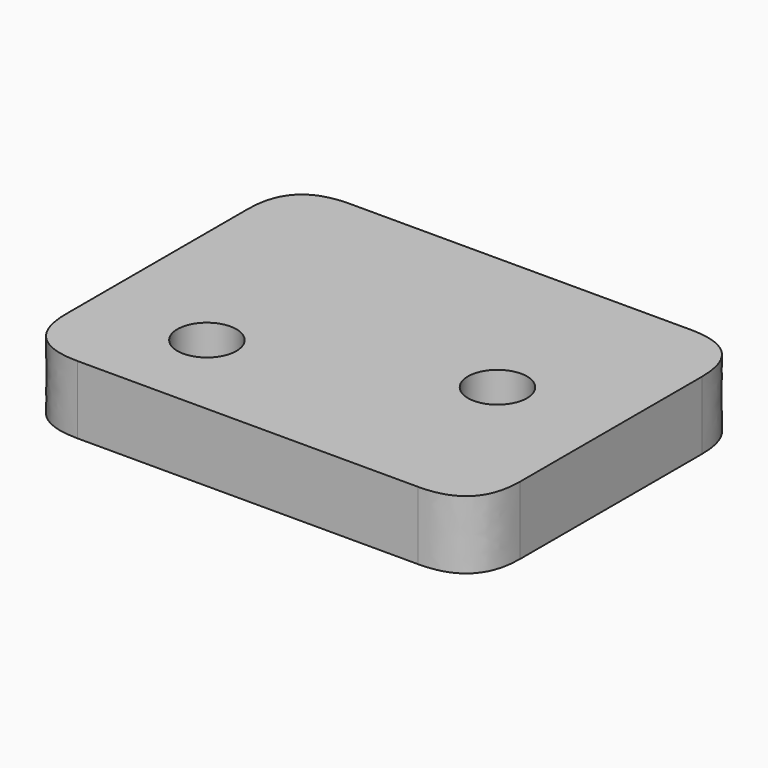
from build123d import *

# Parameters (mm, degrees)
F0_W        = 40
F0_H        = 30
F0_R        = 2.6
F1_DEPTH    = 6
F2_T1_DEPTH = 31


# Not quite as in the source:
# - a fillet or chamfer that OpenCascade refuses, or shapes differently, is made with other operations: its cross-section is extruded or revolved along the edge and cut away or added


with BuildPart() as f1:
    # F0 (on Top) → F1 (new body)
    with BuildSketch(Plane.XY):
        Rectangle(F0_W, F0_H)
        with Locations((-10, -7)):
            Circle(F0_R, mode=Mode.SUBTRACT)
        with Locations((10, 0)):
            Circle(F0_R, mode=Mode.SUBTRACT)
    extrude(amount=F1_DEPTH)

    # F2: fillet of radius 5 on 4 edges, made by hand

    # F2_s2 → F2_t1 (cut)
    with BuildSketch(Plane.XY.offset(-12.5)):
        with BuildLine():
            add(Edge.make_bspline(
                [(-20, -10), (-20, -15), (-15, -15)],
                knots=[0, 0, 0, 1, 1, 1], degree=2, weights=[1, 1, 1]))
            Line((-15, -15), (-20, -15))
            Line((-20, -15), (-20, -10))
        make_face()
        with BuildLine():
            add(Edge.make_bspline(
                [(15, -15), (20, -15), (20, -10)],
                knots=[0, 0, 0, 1, 1, 1], degree=2, weights=[1, 1, 1]))
            Line((20, -10), (20, -15))
            Line((20, -15), (15, -15))
        make_face()
        with BuildLine():
            add(Edge.make_bspline(
                [(15, 15), (20, 15), (20, 10)],
                knots=[0, 0, 0, 1, 1, 1], degree=2, weights=[1, 1, 1]))
            Line((20, 10), (20, 15))
            Line((20, 15), (15, 15))
        make_face()
        with BuildLine():
            add(Edge.make_bspline(
                [(-15, 15), (-20, 15), (-20, 10)],
                knots=[0, 0, 0, 1, 1, 1], degree=2, weights=[1, 1, 1]))
            Line((-20, 10), (-20, 15))
            Line((-20, 15), (-15, 15))
        make_face()
    extrude(amount=F2_T1_DEPTH, mode=Mode.SUBTRACT)


solid = f1.part
